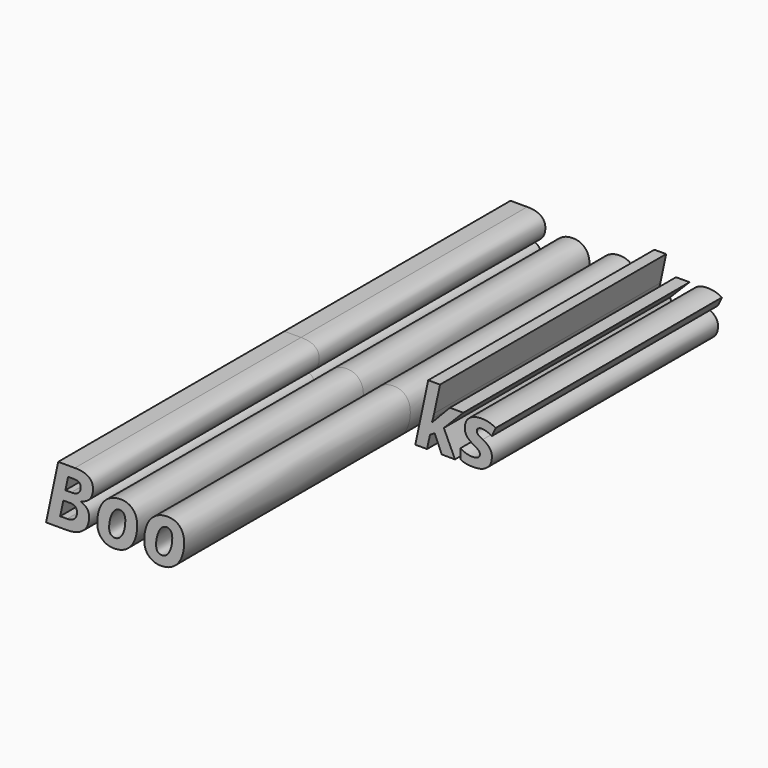
from build123d import *

# Parameters (mm, degrees)
F0_TEXT_SIZE = 7.2103976789
F1_DEPTH     = 25.4
F2_DEPTH     = 25.4


# Not quite as in the source:
# - Text() gives the source's letters only with a copy of the font that has no kerning and outlines rounded to 1/6400 em; it was checked with that copy


with BuildPart() as f1:
    # F0 (on Front) → F1 (new body)
    with BuildSketch(Plane.XZ):
        with Locations((-54.2052462697, 48.0976179242)):
            Text('Books', F0_TEXT_SIZE, font='Open Sans', font_style=FontStyle.BOLDITALIC, text_align=(TextAlign.LEFT, TextAlign.BOTTOM))
    extrude(amount=F1_DEPTH)


with BuildPart() as f2:
    # F2 (new): a face of the model
    f2_faces = [f1.part.faces().sort_by_distance(p)[0] for p in [
        (-49.3626052821, -25.4, 49.5793992801),
    ]]
    extrude(f2_faces, amount=F2_DEPTH)


with BuildPart() as f2b:
    # F2#2 (new): a face of the model
    f2_2_faces = [f1.part.faces().sort_by_distance(p)[0] for p in [
        (-51.8754475215, -25.4, 50.635866292),
    ]]
    extrude(f2_2_faces, amount=F2_DEPTH)


with BuildPart() as f2c:
    # F2#3 (new): a face of the model
    f2_3_faces = [f1.part.faces().sort_by_distance(p)[0] for p in [
        (-45.1445226399, -25.4, 49.5793992801),
    ]]
    extrude(f2_3_faces, amount=F2_DEPTH)


solid = Compound([f1.part, f2.part, f2b.part, f2c.part])
